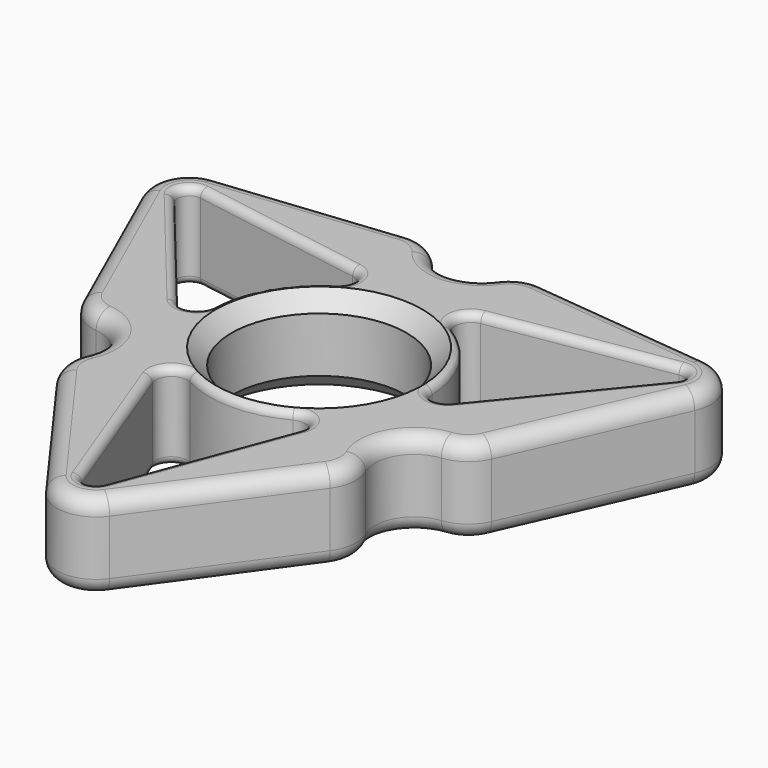
from build123d import *

# Parameters (mm, degrees)
F1_DEPTH = 11
F2_R     = 11.15
F3_DEPTH = 11.001
F4_R     = 5
F6_DEPTH = 11.001
F8_R     = 2
F9_DEPTH = 11.0010001
F10_R    = 1


# Not quite as in the source:
# - a fillet or chamfer that OpenCascade refuses, or shapes differently, is made with other operations: its cross-section is extruded or revolved along the edge and cut away or added


with BuildPart() as f1:
    # F0 (on Top) → F1 (new body)
    with BuildSketch(Plane.XY):
        Polygon((0, 26), (-38.1051177665, 22), (38.1051177665, 22), align=None)
        Polygon((38.1051177665, 22), (-38.1051177665, 22), (0, -44), align=None)
        Polygon((0, -44), (-38.1051177665, 22), (-22.5166604984, -13), align=None)
        Polygon((22.5166604984, -13), (38.1051177665, 22), (0, -44), align=None)
    extrude(amount=F1_DEPTH)

    # F2 (on face) → F3 (cut, through all)
    with BuildSketch(Plane.XY.offset(11)):
        Circle(F2_R)
    extrude(amount=-F3_DEPTH, mode=Mode.SUBTRACT)

    # F4
    f4_edges = [f1.edges().sort_by_distance(p)[0] for p in [
        (0, -44, 5.5),
        (-38.105118, 22, 5.5),
        (38.105118, 22, 5.5),
    ]]
    fillet(f4_edges, radius=F4_R)

    # F5 (on face) → F6 (cut, through all)
    with BuildSketch(Plane.XY.offset(11)):
        with BuildLine():
            ThreePointArc((-8.612929891, 25.095876838), (-6.0566570255, 24.6906622679), (-4.04546707, 23.0615997234))
            ThreePointArc((-4.04546707, 23.0615997234), (0, 21), (4.04546707, 23.0615997234))
            ThreePointArc((4.04546707, 23.0615997234), (6.0566570255, 24.6906622679), (8.612929891, 25.095876838))
            Line((8.612929891, 25.095876838), (0, 26))
            Line((0, 26), (-8.612929891, 25.095876838))
        make_face()
        with BuildLine():
            Line((-22.5166604984, -13), (-17.4272019264, -20.0069545056))
            ThreePointArc((-17.4272019264, -20.0069545056), (-18.3544122475, -17.5905499801), (-17.9491976774, -15.0342771145))
            ThreePointArc((-17.9491976774, -15.0342771145), (-18.1865334795, -10.5), (-21.9946647474, -8.0273226089))
            ThreePointArc((-21.9946647474, -8.0273226089), (-24.411069273, -7.1001122878), (-26.0401318175, -5.0889223323))
            Line((-26.0401318175, -5.0889223323), (-22.5166604984, -13))
        make_face()
        with BuildLine():
            Line((22.5166604984, -13), (26.0401318175, -5.0889223323))
            ThreePointArc((26.0401318175, -5.0889223323), (24.411069273, -7.1001122878), (21.9946647474, -8.0273226089))
            ThreePointArc((21.9946647474, -8.0273226089), (18.1865334795, -10.5), (17.9491976774, -15.0342771145))
            ThreePointArc((17.9491976774, -15.0342771145), (18.3544122475, -17.5905499801), (17.4272019264, -20.0069545056))
            Line((17.4272019264, -20.0069545056), (22.5166604984, -13))
        make_face()
    extrude(amount=-F6_DEPTH, mode=Mode.SUBTRACT)

    # F8
    f8_edges = [f1.edges().sort_by_distance(p)[0] for p in [
        (-35.067074, 20.245985, 0),
        (-31.258943, 22.718662, 5.5),
        (-35.30441, 15.711707, 5.5),
        (-35.067074, 20.245985, 11),
        (-30.672271, 5.311393, 0),
        (-26.040132, -5.088922, 5.5),
        (-30.672271, 5.311393, 11),
        (-24.411069, -7.100112, 11),
        (-24.411069, -7.100112, 0),
        (-21.994665, -8.027323, 5.5),
        (-18.186533, -10.5, 11),
        (-18.186533, -10.5, 0),
        (-17.949198, -15.034277, 5.5),
        (-18.354412, -17.59055, 11),
        (-18.354412, -17.59055, 0),
        (-17.427202, -20.006955, 5.5),
        (-10.736334, -29.218662, 0),
        (-4.045467, -38.430369, 5.5),
        (-10.736334, -29.218662, 11),
        (0, -40.491969, 0),
        (4.045467, -38.430369, 5.5),
        (0, -40.491969, 11),
        (10.736334, -29.218662, 0),
        (17.427202, -20.006955, 5.5),
        (10.736334, -29.218662, 11),
        (18.354412, -17.59055, 11),
        (18.354412, -17.59055, 0),
        (17.949198, -15.034277, 5.5),
        (18.186533, -10.5, 11),
        (18.186533, -10.5, 0),
        (21.994665, -8.027323, 5.5),
        (24.411069, -7.100112, 11),
        (24.411069, -7.100112, 0),
        (26.040132, -5.088922, 5.5),
        (30.672271, 5.311393, 0),
        (35.30441, 15.711707, 5.5),
        (30.672271, 5.311393, 11),
        (35.067074, 20.245985, 0),
        (31.258943, 22.718662, 5.5),
        (35.067074, 20.245985, 11),
        (19.935936, 23.907269, 0),
        (8.61293, 25.095877, 5.5),
        (19.935936, 23.907269, 11),
        (6.056657, 24.690662, 11),
        (6.056657, 24.690662, 0),
        (4.045467, 23.0616, 5.5),
        (0, 21, 11),
        (0, 21, 0),
        (-4.045467, 23.0616, 5.5),
        (-6.056657, 24.690662, 11),
        (-6.056657, 24.690662, 0),
        (-8.61293, 25.095877, 5.5),
        (-19.935936, 23.907269, 0),
        (-19.935936, 23.907269, 11),
    ]]
    fillet(f8_edges, radius=F8_R)

    # F7 (on face) → F9 (cut, through all)
    with BuildSketch(Plane.XY.offset(11)):
        with BuildLine():
            Line((-9.3757335028, -14.8356200168), (-1.4038914618, -36.020257742))
            ThreePointArc((-1.4038914618, -36.020257742), (0, -36.991969219), (1.4038914618, -36.020257742))
            Line((1.4038914618, -36.020257742), (9.3757335028, -14.8356200168))
            ThreePointArc((9.3757335028, -14.8356200168), (8.8245705538, -12.6293126314), (6.5658934429, -12.3648309045))
            ThreePointArc((6.5658934429, -12.3648309045), (0, -14), (-6.5658934429, -12.3648309045))
            ThreePointArc((-6.5658934429, -12.3648309045), (-8.8245705538, -12.6293126314), (-9.3757335028, -14.8356200168))
        make_face()
        with BuildLine():
            ThreePointArc((7.4253109553, 11.8686459724), (12.124355653, 7), (13.9912043982, 0.4961849321))
            ThreePointArc((13.9912043982, 0.4961849321), (15.3495908481, -1.3276459614), (17.5358905669, -0.7018133841))
            Line((17.5358905669, -0.7018133841), (31.8964039863, 16.794323201))
            ThreePointArc((31.8964039863, 16.794323201), (32.0359850796, 18.4959846095), (30.4925125246, 19.2259345411))
            Line((30.4925125246, 19.2259345411), (8.1601570641, 15.537433401))
            ThreePointArc((8.1601570641, 15.537433401), (6.5250202942, 13.9569585928), (7.4253109553, 11.8686459724))
        make_face()
        with BuildLine():
            ThreePointArc((-13.9912043982, 0.4961849321), (-12.124355653, 7), (-7.4253109553, 11.8686459724))
            ThreePointArc((-7.4253109553, 11.8686459724), (-6.5250202942, 13.9569585928), (-8.1601570641, 15.537433401))
            Line((-8.1601570641, 15.537433401), (-30.4925125246, 19.2259345411))
            ThreePointArc((-30.4925125246, 19.2259345411), (-32.0359850796, 18.4959846095), (-31.8964039863, 16.794323201))
            Line((-31.8964039863, 16.794323201), (-17.5358905669, -0.7018133841))
            ThreePointArc((-17.5358905669, -0.7018133841), (-15.3495908481, -1.3276459614), (-13.9912043982, 0.4961849321))
        make_face()
    extrude(amount=-F9_DEPTH, mode=Mode.SUBTRACT)

    # F10
    f10_edges = [f1.edges().sort_by_distance(p)[0] for p in [
        (32.035985, 18.495985, 11),
        (30.492513, 19.225935, 5.5),
        (32.035985, 18.495985, 0),
        (31.896404, 16.794323, 5.5),
        (19.326335, 17.381684, 11),
        (8.160157, 15.537433, 5.5),
        (19.326335, 17.381684, 0),
        (-19.326335, 17.381684, 11),
        (-30.492513, 19.225935, 5.5),
        (-19.326335, 17.381684, 0),
        (-8.160157, 15.537433, 5.5),
        (-6.52502, 13.956959, 11),
        (-6.52502, 13.956959, 0),
        (-7.425311, 11.868646, 5.5),
        (-12.124356, 7, 11),
        (-12.124356, 7, 0),
        (-13.991204, 0.496185, 5.5),
        (24.716147, 8.046255, 11),
        (24.716147, 8.046255, 0),
        (17.535891, -0.701813, 5.5),
        (0, -14, 11),
        (-6.565893, -12.364831, 5.5),
        (0, -14, 0),
        (6.565893, -12.364831, 5.5),
        (8.824571, -12.629313, 11),
        (8.824571, -12.629313, 0),
        (9.375734, -14.83562, 5.5),
        (5.389812, -25.427939, 11),
        (5.389812, -25.427939, 0),
        (1.403891, -36.020258, 5.5),
        (-24.716147, 8.046255, 11),
        (-17.535891, -0.701813, 5.5),
        (-24.716147, 8.046255, 0),
        (-31.896404, 16.794323, 5.5),
        (12.124356, 7, 11),
        (13.991204, 0.496185, 5.5),
        (12.124356, 7, 0),
        (7.425311, 11.868646, 5.5),
        (6.52502, 13.956959, 11),
        (6.52502, 13.956959, 0),
        (-5.389812, -25.427939, 11),
        (-1.403891, -36.020258, 5.5),
        (-5.389812, -25.427939, 0),
        (-9.375734, -14.83562, 5.5),
        (-32.035985, 18.495985, 11),
        (-32.035985, 18.495985, 0),
        (-8.824571, -12.629313, 11),
        (-8.824571, -12.629313, 0),
        (-15.349591, -1.327646, 11),
        (-15.349591, -1.327646, 0),
        (15.349591, -1.327646, 11),
        (15.349591, -1.327646, 0),
        (0, -36.991969, 11),
        (0, -36.991969, 0),
    ]]
    fillet(f10_edges, radius=F10_R)

    # F11: chamfer of 2 on 3 edges, made by hand

    # F11_s1 → F11_t2 (revolve, cut)
    with BuildSketch(Plane.XZ):
        Polygon((13.15, 11), (11.15, 9), (11.15, 11), align=None)
    revolve(axis=Axis((0, 0, 11), (0, 0, 1)), mode=Mode.SUBTRACT)

    # F11_s3 → F11_t4 (revolve, cut)
    with BuildSketch(Plane.XZ):
        Polygon((11.15, 2), (13.15, 0), (11.15, 0), align=None)
    revolve(axis=Axis((0, 0, 0), (0, 0, 1)), mode=Mode.SUBTRACT)


solid = f1.part
